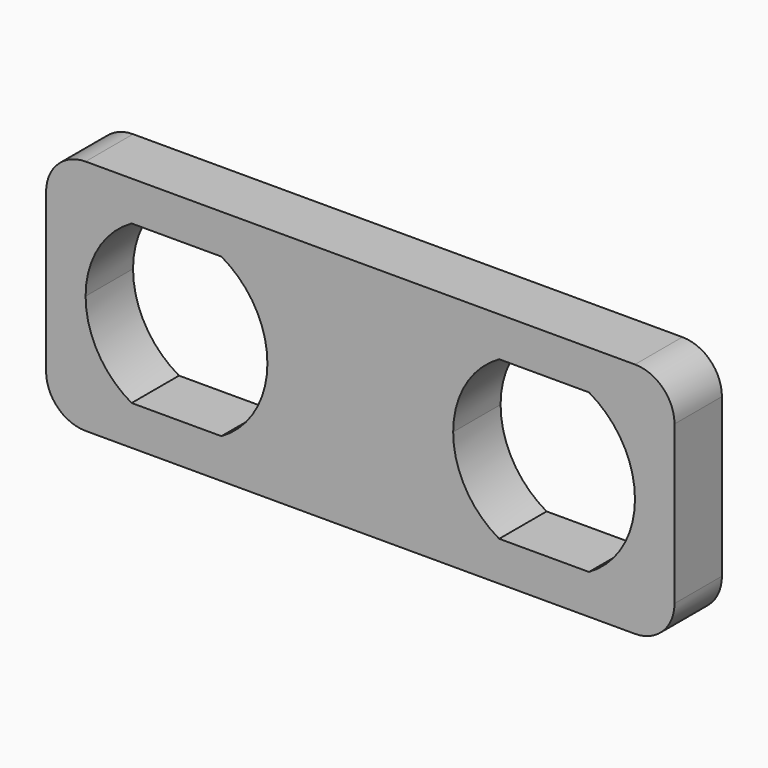
from build123d import *

# Parameters (mm, degrees)
F0_TEXT_SIZE = 13.3411163309
F1_DEPTH     = 7.5
F2_R         = 5


# Not quite as in the source:
# - Text() gives the source's letters only with a copy of the font that has no kerning and outlines rounded to 1/6400 em; it was checked with that copy


with BuildPart() as f1:
    # F0 (on Front) → F1 (new body)
    with BuildSketch(Plane.XZ):
        with BuildLine():
            Line((-35, 0), (-11.5, 0))
            ThreePointArc((-11.5, 0), (-9.9387485625, 5.785436631), (-5.6789083458, 10))
            ThreePointArc((-5.6789083458, 10), (0, 11.5), (5.6789083458, 10))
            ThreePointArc((5.6789083458, 10), (9.9387485625, 5.785436631), (11.5, 0))
            Line((11.5, 0), (16.5, 0))
            Line((16.5, 0), (16.5, 15))
            Line((16.5, 15), (-63, 15))
            Line((-63, 15), (-63, 0))
            Line((-63, 0), (-58, 0))
            ThreePointArc((-58, 0), (-56.4387485625, 5.785436631), (-52.1789083458, 10))
            ThreePointArc((-52.1789083458, 10), (-46.5, 11.5), (-40.8210916542, 10))
            ThreePointArc((-40.8210916542, 10), (-36.5612514375, 5.785436631), (-35, 0))
        make_face()
        with BuildLine():
            Line((-27.7581276666, 4.7613837399), (-27.7581276666, 3.7587154657))
            Line((-27.7581276666, 3.7587154657), (-34.0180295949, 3.7587154657))
            Line((-34.0180295949, 3.7587154657), (-34.0180295949, 4.6905090594))
            Line((-34.0180295949, 4.6905090594), (-31.5103166346, 7.2107293163))
            add(Edge.make_bspline(
                [(-31.5103166346, 7.2107293163), (-30.3638144499, 8.371823347), (-29.9990183003, 8.8669038358)],
                knots=[0, 0, 0, 1, 1, 1], degree=2))
            add(Edge.make_bspline(
                [(-29.9990183003, 8.8669038358), (-29.6342221506, 9.3619843246), (-29.4518240757, 9.8310079456)],
                knots=[0, 0, 0, 1, 1, 1], degree=2))
            add(Edge.make_bspline(
                [(-29.4518240757, 9.8310079456), (-29.2694260009, 10.3000315667), (-29.2694260009, 10.8399298682)],
                knots=[0, 0, 0, 1, 1, 1], degree=2))
            add(Edge.make_bspline(
                [(-29.2694260009, 10.8399298682), (-29.2694260009, 11.6028749583), (-29.7321959736, 12.0489685357)],
                knots=[0, 0, 0, 1, 1, 1], degree=2))
            add(Edge.make_bspline(
                [(-29.7321959736, 12.0489685357), (-30.1949659464, 12.495062113), (-31.0162784205, 12.495062113)],
                knots=[0, 0, 0, 1, 1, 1], degree=2))
            add(Edge.make_bspline(
                [(-31.0162784205, 12.495062113), (-31.6082904577, 12.495062113), (-32.1398505615, 12.2991144669)],
                knots=[0, 0, 0, 1, 1, 1], degree=2))
            add(Edge.make_bspline(
                [(-32.1398505615, 12.2991144669), (-32.6714106653, 12.1031668208), (-33.3217900864, 11.5882831124)],
                knots=[0, 0, 0, 1, 1, 1], degree=2))
            Line((-33.3217900864, 11.5882831124), (-33.8950411788, 12.32412906))
            add(Edge.make_bspline(
                [(-33.8950411788, 12.32412906), (-32.5796904905, 13.418517509), (-31.0287857171, 13.418517509)],
                knots=[0, 0, 0, 1, 1, 1], degree=2))
            add(Edge.make_bspline(
                [(-31.0287857171, 13.418517509), (-29.6863358863, 13.418517509), (-28.9244330708, 12.7316584729)],
                knots=[0, 0, 0, 1, 1, 1], degree=2))
            add(Edge.make_bspline(
                [(-28.9244330708, 12.7316584729), (-28.1625302553, 12.0447994368), (-28.1625302553, 10.8857899556)],
                knots=[0, 0, 0, 1, 1, 1], degree=2))
            add(Edge.make_bspline(
                [(-28.1625302553, 10.8857899556), (-28.1625302553, 9.9790109549), (-28.6711603154, 9.0930774486)],
                knots=[0, 0, 0, 1, 1, 1], degree=2))
            add(Edge.make_bspline(
                [(-28.6711603154, 9.0930774486), (-29.1797903756, 8.2071439422), (-30.5722693926, 6.8521868149)],
                knots=[0, 0, 0, 1, 1, 1], degree=2))
            Line((-30.5722693926, 6.8521868149), (-32.6568188193, 4.8134974756))
            Line((-32.6568188193, 4.8134974756), (-32.6568188193, 4.7613837399))
            Line((-32.6568188193, 4.7613837399), (-27.7581276666, 4.7613837399))
        make_face(mode=Mode.SUBTRACT)
        with BuildLine():
            add(Edge.make_bspline(
                [(-24.9064640508, 9.4266053569), (-24.1581108066, 9.5766929156), (-23.4139266613, 9.5766929156)],
                knots=[0, 0, 0, 1, 1, 1], degree=2))
            add(Edge.make_bspline(
                [(-23.4139266613, 9.5766929156), (-21.9088819752, 9.5766929156), (-21.0458785126, 8.8304242208)],
                knots=[0, 0, 0, 1, 1, 1], degree=2))
            add(Edge.make_bspline(
                [(-21.0458785126, 8.8304242208), (-20.1828750499, 8.0841555261), (-20.1828750499, 6.7875657827)],
                knots=[0, 0, 0, 1, 1, 1], degree=2))
            add(Edge.make_bspline(
                [(-20.1828750499, 6.7875657827), (-20.1828750499, 5.3096202391), (-21.1240491161, 4.4685045455)],
                knots=[0, 0, 0, 1, 1, 1], degree=2))
            add(Edge.make_bspline(
                [(-21.1240491161, 4.4685045455), (-22.0652231822, 3.6273888518), (-23.720355427, 3.6273888518)],
                knots=[0, 0, 0, 1, 1, 1], degree=2))
            add(Edge.make_bspline(
                [(-23.720355427, 3.6273888518), (-25.3296275844, 3.6273888518), (-26.1759546517, 4.1422725602)],
                knots=[0, 0, 0, 1, 1, 1], degree=2))
            Line((-26.1759546517, 4.1422725602), (-26.1759546517, 5.1845472735))
            add(Edge.make_bspline(
                [(-26.1759546517, 5.1845472735), (-25.7215228767, 4.8927103538), (-25.044044313, 4.7259463997)],
                knots=[0, 0, 0, 1, 1, 1], degree=2))
            add(Edge.make_bspline(
                [(-25.044044313, 4.7259463997), (-24.3665657493, 4.5591824455), (-23.7078481305, 4.5591824455)],
                knots=[0, 0, 0, 1, 1, 1], degree=2))
            add(Edge.make_bspline(
                [(-23.7078481305, 4.5591824455), (-22.5613459458, 4.5591824455), (-21.9266006454, 5.1001230217)],
                knots=[0, 0, 0, 1, 1, 1], degree=2))
            add(Edge.make_bspline(
                [(-21.9266006454, 5.1001230217), (-21.2918553449, 5.641063598), (-21.2918553449, 6.6645773665)],
                knots=[0, 0, 0, 1, 1, 1], degree=2))
            add(Edge.make_bspline(
                [(-21.2918553449, 6.6645773665), (-21.2918553449, 8.6574066184), (-23.7328627236, 8.6574066184)],
                knots=[0, 0, 0, 1, 1, 1], degree=2))
            add(Edge.make_bspline(
                [(-23.7328627236, 8.6574066184), (-24.3519739033, 8.6574066184), (-25.3879949684, 8.4677126206)],
                knots=[0, 0, 0, 1, 1, 1], degree=2))
            Line((-25.3879949684, 8.4677126206), (-25.9487387642, 8.826255122))
            Line((-25.9487387642, 8.826255122), (-25.5901962628, 13.2830217963))
            Line((-25.5901962628, 13.2830217963), (-20.8540999653, 13.2830217963))
            Line((-20.8540999653, 13.2830217963), (-20.8540999653, 12.2866071703))
            Line((-20.8540999653, 12.2866071703), (-24.6646563173, 12.2866071703))
            Line((-24.6646563173, 12.2866071703), (-24.9064640508, 9.4266053569))
        make_face(mode=Mode.SUBTRACT)
        with BuildLine():
            add(Edge.make_bspline(
                [(-12.8942479795, 11.4684215203), (-12.5033949619, 10.5147401576), (-12.5033949619, 9.2181504142)],
                knots=[0, 0, 0, 1, 1, 1], degree=2))
            add(Edge.make_bspline(
                [(-12.5033949619, 9.2181504142), (-12.5033949619, 3.6273888518), (-16.8288350224, 3.6273888518)],
                knots=[0, 0, 0, 1, 1, 1], degree=2))
            add(Edge.make_bspline(
                [(-16.8288350224, 3.6273888518), (-17.5855264642, 3.6273888518), (-18.0274509427, 3.7587154657)],
                knots=[0, 0, 0, 1, 1, 1], degree=2))
            Line((-18.0274509427, 3.7587154657), (-18.0274509427, 4.6905090594))
            add(Edge.make_bspline(
                [(-18.0274509427, 4.6905090594), (-17.506313586, 4.5216605558), (-16.8434268683, 4.5216605558)],
                knots=[0, 0, 0, 1, 1, 1], degree=2))
            add(Edge.make_bspline(
                [(-16.8434268683, 4.5216605558), (-15.2800147983, 4.5216605558), (-14.4816323679, 5.4888914898)],
                knots=[0, 0, 0, 1, 1, 1], degree=2))
            add(Edge.make_bspline(
                [(-14.4816323679, 5.4888914898), (-13.6832499375, 6.4561224238), (-13.6123752569, 8.455205324)],
                knots=[0, 0, 0, 1, 1, 1], degree=2))
            Line((-13.6123752569, 8.455205324), (-13.6895035857, 8.455205324))
            add(Edge.make_bspline(
                [(-13.6895035857, 8.455205324), (-14.0480460871, 7.9153070225), (-14.641100399, 7.6318083005)],
                knots=[0, 0, 0, 1, 1, 1], degree=2))
            add(Edge.make_bspline(
                [(-14.641100399, 7.6318083005), (-15.2341547109, 7.3483095784), (-15.9762543068, 7.3483095784)],
                knots=[0, 0, 0, 1, 1, 1], degree=2))
            add(Edge.make_bspline(
                [(-15.9762543068, 7.3483095784), (-17.2394912594, 7.3483095784), (-17.98263313, 8.1039587456)],
                knots=[0, 0, 0, 1, 1, 1], degree=2))
            add(Edge.make_bspline(
                [(-17.98263313, 8.1039587456), (-18.7257750007, 8.8596079128), (-18.7257750007, 10.2145650402)],
                knots=[0, 0, 0, 1, 1, 1], degree=2))
            add(Edge.make_bspline(
                [(-18.7257750007, 10.2145650402), (-18.7257750007, 11.698764232), (-17.8950820541, 12.5586408705)],
                knots=[0, 0, 0, 1, 1, 1], degree=2))
            add(Edge.make_bspline(
                [(-17.8950820541, 12.5586408705), (-17.0643891076, 13.418517509), (-15.7094319802, 13.418517509)],
                knots=[0, 0, 0, 1, 1, 1], degree=2))
            add(Edge.make_bspline(
                [(-15.7094319802, 13.418517509), (-14.7380319474, 13.418517509), (-14.0115664722, 12.920310196)],
                knots=[0, 0, 0, 1, 1, 1], degree=2))
            add(Edge.make_bspline(
                [(-14.0115664722, 12.920310196), (-13.285100997, 12.422102883), (-12.8942479795, 11.4684215203)],
                knots=[0, 0, 0, 1, 1, 1], degree=2))
        make_face(mode=Mode.SUBTRACT)
        with BuildLine():
            ThreePointArc((-5.6789083458, -10), (-9.9387485625, -5.785436631), (-11.5, 0))
            Line((-11.5, 0), (-35, 0))
            ThreePointArc((-35, 0), (-36.5612514375, -5.785436631), (-40.8210916542, -10))
            ThreePointArc((-40.8210916542, -10), (-46.5, -11.5), (-52.1789083458, -10))
            ThreePointArc((-52.1789083458, -10), (-56.4387485625, -5.785436631), (-58, 0))
            Line((-58, 0), (-63, 0))
            Line((-63, 0), (-63, -15))
            Line((-63, -15), (16.5, -15))
            Line((16.5, -15), (16.5, 0))
            Line((16.5, 0), (11.5, 0))
            ThreePointArc((11.5, 0), (9.9387485625, -5.785436631), (5.6789083458, -10))
            ThreePointArc((5.6789083458, -10), (0, -11.5), (-5.6789083458, -10))
        make_face()
        with Locations((-34.6704935655, 3.7587154657)):
            Text('259', F0_TEXT_SIZE, font='Open Sans', text_align=(TextAlign.LEFT, TextAlign.BOTTOM))
        with BuildLine():
            add(Edge.make_bspline(
                [(-14.6119167071, 12.1625764794), (-15.0903208005, 12.495062113), (-15.7094319802, 12.495062113)],
                knots=[0, 0, 0, 1, 1, 1], degree=2))
            add(Edge.make_bspline(
                [(-15.7094319802, 12.495062113), (-16.6412255739, 12.495062113), (-17.1488133594, 11.8957541528)],
                knots=[0, 0, 0, 1, 1, 1], degree=2))
            add(Edge.make_bspline(
                [(-17.1488133594, 11.8957541528), (-17.6564011448, 11.2964461926), (-17.6564011448, 10.2270723367)],
                knots=[0, 0, 0, 1, 1, 1], degree=2))
            add(Edge.make_bspline(
                [(-17.6564011448, 10.2270723367), (-17.6564011448, 9.2890250947), (-17.1873775237, 8.7522536173)],
                knots=[0, 0, 0, 1, 1, 1], degree=2))
            add(Edge.make_bspline(
                [(-17.1873775237, 8.7522536173), (-16.7183539027, 8.21548214), (-15.7615457159, 8.21548214)],
                knots=[0, 0, 0, 1, 1, 1], degree=2))
            add(Edge.make_bspline(
                [(-15.7615457159, 8.21548214), (-15.1674491293, 8.21548214), (-14.6692418163, 8.4562475987)],
                knots=[0, 0, 0, 1, 1, 1], degree=2))
            add(Edge.make_bspline(
                [(-14.6692418163, 8.4562475987), (-14.1710345033, 8.6970130575), (-13.8844089571, 9.1139229429)],
                knots=[0, 0, 0, 1, 1, 1], degree=2))
            add(Edge.make_bspline(
                [(-13.8844089571, 9.1139229429), (-13.597783411, 9.5308328282), (-13.597783411, 9.9873491527)],
                knots=[0, 0, 0, 1, 1, 1], degree=2))
            add(Edge.make_bspline(
                [(-13.597783411, 9.9873491527), (-13.597783411, 10.6710813646), (-13.8656480123, 11.2505861052)],
                knots=[0, 0, 0, 1, 1, 1], degree=2))
            add(Edge.make_bspline(
                [(-13.8656480123, 11.2505861052), (-14.1335126136, 11.8300908459), (-14.6119167071, 12.1625764794)],
                knots=[0, 0, 0, 1, 1, 1], degree=2))
        make_face()
        with BuildLine():
            ThreePointArc((5.6789083458, 10), (0, 11.5), (-5.6789083458, 10))
            Line((-5.6789083458, 10), (5.6789083458, 10))
        make_face()
        with BuildLine():
            Line((5.6789083458, -10), (-5.6789083458, -10))
            ThreePointArc((-5.6789083458, -10), (0, -11.5), (5.6789083458, -10))
        make_face()
        with BuildLine():
            ThreePointArc((-52.1789083458, -10), (-46.5, -11.5), (-40.8210916542, -10))
            Line((-40.8210916542, -10), (-46.5, -10))
            Line((-46.5, -10), (-52.1789083458, -10))
        make_face()
        with BuildLine():
            Line((-46.5, 10), (-40.8210916542, 10))
            ThreePointArc((-40.8210916542, 10), (-46.5, 11.5), (-52.1789083458, 10))
            Line((-52.1789083458, 10), (-46.5, 10))
        make_face()
    extrude(amount=F1_DEPTH)

    # F2
    f2_edges = [f1.edges().sort_by_distance(p)[0] for p in [
        (-63, -3.75, -15),
        (-63, -3.75, 15),
        (16.5, -3.75, -15),
        (16.5, -3.75, 15),
    ]]
    fillet(f2_edges, radius=F2_R)


solid = f1.part
